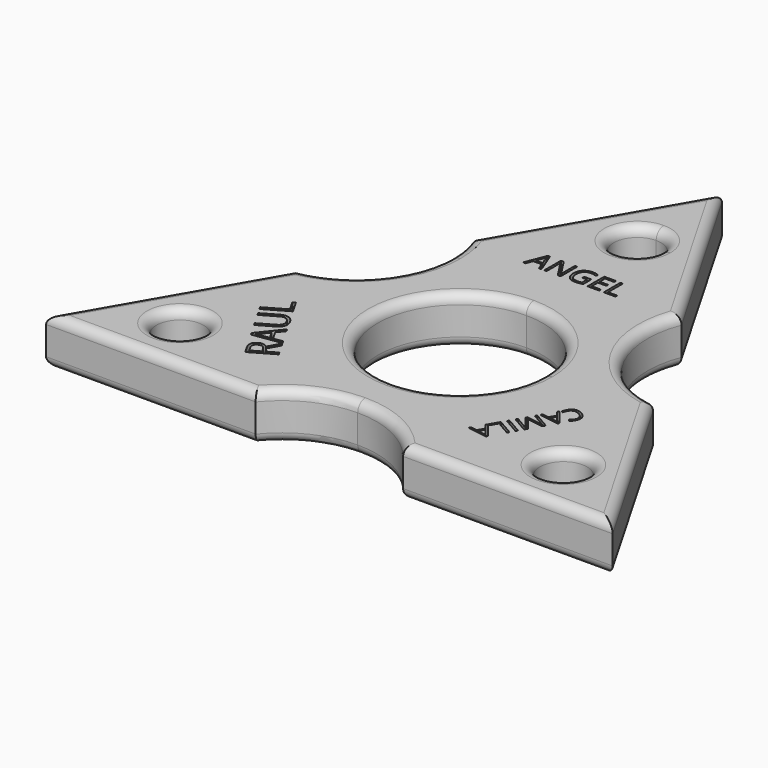
from build123d import *

# Parameters (mm, degrees)
F0_R           = 3.175
F1_DEPTH       = 3.175
F1_DEPTH_BACK  = 3.175
F2_R           = 1.27
F3_R           = 1.27
F4_TEXT_SIZE   = 3.929797
F6_DEPTH       = 3.556
F6_DEPTH_BACK  = 3.556
F5_TEXT_SIZE   = 5.000308
F7_DEPTH       = 3.556
F7_DEPTH_BACK  = 3.556
F8_DEPTH       = 3.556
F9_DEPTH       = 3.556
F10_TEXT_SIZE  = 3.468021
F11_DEPTH      = 3.556
F11_DEPTH_BACK = 3.556
F12_DEPTH      = 3.556


# Not quite as in the source:
# - Text() gives the source's letters only with a copy of the font that has no kerning and outlines rounded to 1/6400 em; it was checked with that copy


with BuildPart() as f1:
    # F0 (on Top) → F1 (new body, two sides)
    with BuildSketch(Plane.XY) as f1_sk:
        with BuildLine():
            Line((-38.1, -24.214669), (-9.915484, -24.214669))
            ThreePointArc((-9.915484, -24.214669), (-5.500379, -20.703145), (0, -19.450233))
            Line((0, -19.450233), (0, -13.330124))
            ThreePointArc((0, -13.330124), (-11.1125, -2.217624), (0, 8.894876))
            Line((0, 8.894876), (0, 24.377467))
            ThreePointArc((0, 24.377467), (-3.175, 27.552467), (0, 30.727467))
            Line((0, 30.727467), (0, 41.776467))
            Line((0, 41.776467), (-14.092258, 17.36796))
            ThreePointArc((-14.092258, 17.36796), (-13.441759, 15.098914), (-13.2224, 12.748681))
            ThreePointArc((-13.2224, 12.748681), (-16.288965, 4.472998), (-24.007742, 0.193838))
            Line((-24.007742, 0.193838), (-38.1, -24.214669))
        make_face()
        with Locations((-25.781655, -17.102669)):
            Circle(F0_R, mode=Mode.SUBTRACT)
        with BuildLine():
            ThreePointArc((0, -19.450233), (5.500379, -20.703145), (9.915484, -24.214669))
            Line((9.915484, -24.214669), (38.1, -24.214669))
            Line((38.1, -24.214669), (24.007742, 0.193838))
            ThreePointArc((24.007742, 0.193838), (14.923878, 6.398681), (14.092258, 17.36796))
            Line((14.092258, 17.36796), (0, 41.776467))
            Line((0, 41.776467), (0, 30.727467))
            ThreePointArc((0, 30.727467), (2.245064, 29.797531), (3.175, 27.552467))
            ThreePointArc((3.175, 27.552467), (2.245064, 25.307403), (0, 24.377467))
            Line((0, 24.377467), (0, 8.894876))
            ThreePointArc((0, 8.894876), (7.857724, 5.6401), (11.1125, -2.217624))
            ThreePointArc((11.1125, -2.217624), (7.857724, -10.075348), (0, -13.330124))
            Line((0, -13.330124), (0, -19.450233))
        make_face()
        with Locations((25.788964, -17.106889)):
            Circle(F0_R, mode=Mode.SUBTRACT)
    extrude(amount=-F1_DEPTH)
    extrude(f1_sk.sketch, amount=F1_DEPTH_BACK)

    # F2
    f2_edges = [f1.edges().sort_by_distance(p)[0] for p in [
        (-14.923878, 6.398681, 3.175),
        (-31.053871, -12.010416, 3.175),
        (-24.007742, -24.214669, 3.175),
        (0, -19.450233, 3.175),
        (24.007742, -24.214669, 3.175),
        (31.053871, -12.010416, 3.175),
        (14.923878, 6.398681, 3.175),
        (7.046129, 29.572213, 3.175),
        (-7.046129, 29.572213, 3.175),
        (0, -13.330124, 3.175),
        (0, 24.377467, 3.175),
        (-28.956655, -17.102669, 3.175),
        (22.613964, -17.106889, 3.175),
    ]]
    fillet(f2_edges, radius=F2_R)

    # F3
    f3_edges = [f1.edges().sort_by_distance(p)[0] for p in [
        (-14.923878, 6.398681, -3.175),
        (-31.053871, -12.010416, -3.175),
        (-24.007742, -24.214669, -3.175),
        (0, -19.450233, -3.175),
        (24.007742, -24.214669, -3.175),
        (31.053871, -12.010416, -3.175),
        (14.923878, 6.398681, -3.175),
        (7.046129, 29.572213, -3.175),
        (-7.046129, 29.572213, -3.175),
        (0, -13.330124, -3.175),
        (0, 24.377467, -3.175),
        (-28.956655, -17.102669, -3.175),
        (22.613964, -17.106889, -3.175),
    ]]
    fillet(f3_edges, radius=F3_R)

    # F4 (on Top) → F6 (join, two sides)
    with BuildSketch(Plane.XY) as f6_sk:
        with Locations((-6.292688, 16.18844)):
            Text('ANGEL', F4_TEXT_SIZE, font='Open Sans', text_align=(TextAlign.LEFT, TextAlign.BOTTOM))
    extrude(amount=-F6_DEPTH)
    extrude(f6_sk.sketch, amount=F6_DEPTH_BACK)

    # F5 (on Top) → F7 (join, two sides)
    with BuildSketch(Plane.XY) as f7_sk:
        with Locations(Location((-13.000399, -16.580712), (0, 0, 120))):
            Text('RAUL', F5_TEXT_SIZE, font='Open Sans', text_align=(TextAlign.LEFT, TextAlign.BOTTOM))
    extrude(amount=-F7_DEPTH)
    extrude(f7_sk.sketch, amount=F7_DEPTH_BACK)

    # F4 (on Top) → F8 (cut)
    with BuildSketch(Plane.XY):
        with Locations((-6.292688, 16.18844)):
            Text('ANGEL', F4_TEXT_SIZE, font='Open Sans', text_align=(TextAlign.LEFT, TextAlign.BOTTOM))
    extrude(amount=F8_DEPTH, mode=Mode.SUBTRACT)

    # F5 (on Top) → F9 (cut)
    with BuildSketch(Plane.XY):
        with Locations(Location((-13.000399, -16.580712), (0, 0, 120))):
            Text('RAUL', F5_TEXT_SIZE, font='Open Sans', text_align=(TextAlign.LEFT, TextAlign.BOTTOM))
    extrude(amount=F9_DEPTH, mode=Mode.SUBTRACT)

    # F10 (on Top) → F11 (join, two sides)
    with BuildSketch(Plane.XY) as f11_sk:
        with Locations(Location((18.983503, -5.958025), (0, 0, -120))):
            Text('CAMILA', F10_TEXT_SIZE, font='Open Sans', text_align=(TextAlign.LEFT, TextAlign.BOTTOM))
    extrude(amount=F11_DEPTH)
    extrude(f11_sk.sketch, amount=-F11_DEPTH_BACK)

    # F10 (on Top) → F12 (cut)
    with BuildSketch(Plane.XY):
        with Locations(Location((18.983503, -5.958025), (0, 0, -120))):
            Text('CAMILA', F10_TEXT_SIZE, font='Open Sans', text_align=(TextAlign.LEFT, TextAlign.BOTTOM))
    extrude(amount=F12_DEPTH, mode=Mode.SUBTRACT)


solid = f1.part
